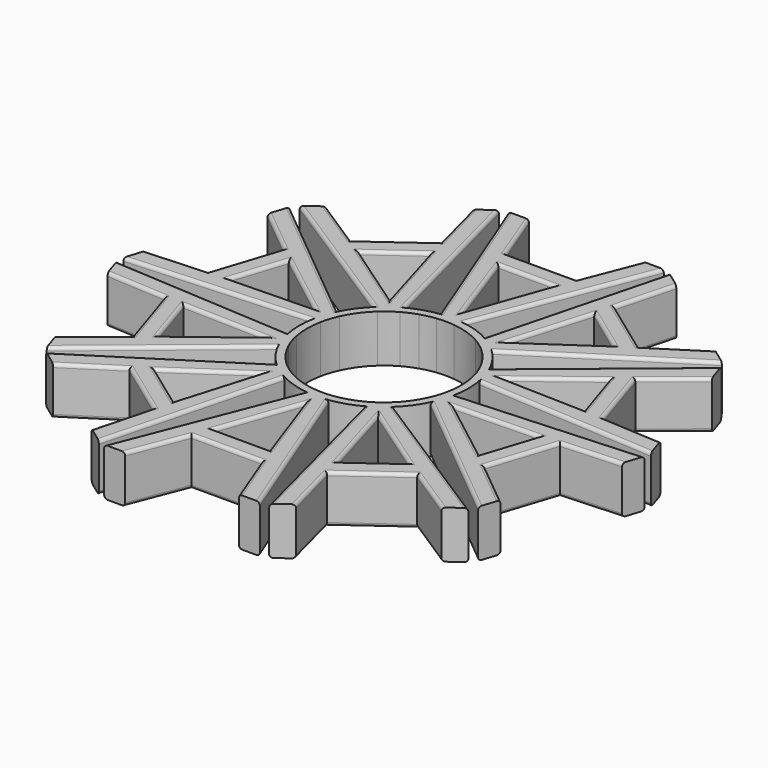
from build123d import *

# Parameters (mm, degrees)
F1_DEPTH = 7
F2_R     = 0.4828427125
F3_COUNT = 10


# Not quite as in the source:
# - a feature names something its author has since deleted; it is built from what else it names


with BuildPart() as f1:
    # F0 (on Top) → F1 (new body)
    with BuildSketch(Plane.XY):
        with BuildLine():
            ThreePointArc((1.3026409259, 11.2246659914), (8.4383008498, 7.5156555781), (11.3, 0))
            ThreePointArc((11.3, 0), (-7.5187570092, -8.4355375073), (-1.2943881482, 11.2256206653))
            Line((-1.2943881482, 11.2256206653), (-1.7251015749, 12.3244931269))
            ThreePointArc((-1.7251015749, 12.3244931269), (-8.167032366, -9.3898183481), (12.4446416693, 0))
            ThreePointArc((12.4446416693, 0), (9.3930845888, 8.1632755794), (1.7349611568, 12.3231090258))
            Line((1.7349611568, 12.3231090258), (1.3026409259, 11.2246659914))
        make_face()
        with BuildLine():
            ThreePointArc((-1.2943881482, 11.2256206653), (0.0041539061, 11.2999992365), (1.3026409259, 11.2246659914))
            Line((1.3026409259, 11.2246659914), (1.7349611568, 12.3231090258))
            ThreePointArc((1.7349611568, 12.3231090258), (0.0049781295, 12.4446406737), (-1.7251015749, 12.3244931269))
            Line((-1.7251015749, 12.3244931269), (-1.2943881482, 11.2256206653))
        make_face()
        with BuildLine():
            ThreePointArc((-1.7251015749, 12.3244931269), (0.0049781295, 12.4446406737), (1.7349611568, 12.3231090258))
            Line((1.7349611568, 12.3231090258), (11.4559943904, 37.0223955251))
            Line((11.4559943904, 37.0223955251), (8.3686571161, 37.0223955251))
            Line((8.3686571161, 37.0223955251), (5.1758160407, 28.8522769697))
            Line((5.1758160407, 28.8522769697), (-5.1490863261, 28.8522769697))
            Line((-5.1490863261, 28.8522769697), (-8.3004653861, 37.0223955251))
            Line((-8.3004653861, 37.0223955251), (-11.4056773891, 37.0223955251))
            Line((-11.4056773891, 37.0223955251), (-1.7251015749, 12.3244931269))
        make_face()
        Polygon((-4.0709860332, 26.0975067504), (4.0977142343, 26.0975067504), (-0.0073703414, 14.5850260742), align=None, mode=Mode.SUBTRACT)
    extrude(amount=F1_DEPTH)

    # F2
    f2_edges = [f1.edges().sort_by_distance(p)[0] for p in [
        (-6.565389, 24.673444, 7),
        (6.595478, 24.672752, 7),
        (6.595478, 24.672752, 0),
        (-6.565389, 24.673444, 0),
        (6.772237, 32.937336, 7),
        (2.045172, 20.341266, 7),
        (-2.039178, 20.341266, 7),
        (-6.724776, 32.937336, 7),
        (0.013364, 26.097507, 7),
        (0.013365, 28.852277, 7),
        (0.013365, 28.852277, 0),
        (0.013364, 26.097507, 0),
        (2.045172, 20.341266, 0),
        (-2.039178, 20.341266, 0),
        (-6.724776, 32.937336, 0),
        (6.772237, 32.937336, 0),
    ]]
    fillet(f2_edges, radius=F2_R)

    # F3: F1 ×10 about axis
    f3_axis = Axis((0, 0, 0), (0, 0, -1))


with BuildPart() as f1_1:
    add(f1.part)
    for i in range(1, F3_COUNT):
        add(f1.part.rotate(f3_axis, i * 360 / F3_COUNT))


solid = f1_1.part
